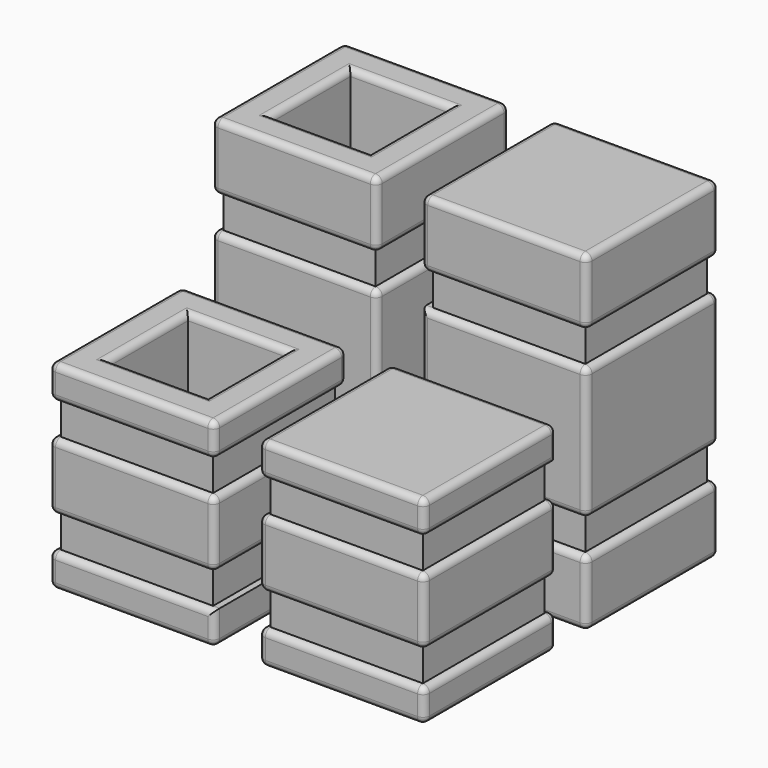
from build123d import *

# Parameters (mm, degrees)
F0_W     = 25
F0_H     = 25
F0_W_2   = 23
F0_H_2   = 23
F0_W_3   = 15
F0_H_3   = 15
F1_DEPTH = 50
F2_DEPTH = 30
F3_START = 20
F3_DEPTH = 5
F4_START = 5
F4_DEPTH = 5
F5_START = 35
F5_DEPTH = 5
F6_START = 10
F6_DEPTH = 5
F7_R     = 0.99999
F7_2_R   = 0.99999
F8_R     = 0.99999
F8_2_R   = 0.99999


# Not quite as in the source:
# - a fillet or chamfer is up to 0.001 mm smaller than in the source, because OpenCascade refuses the exact size


with BuildPart() as f1:
    # F0 (on Top) → F1 (new body)
    with BuildSketch(Plane.XY):
        with Locations((15.8383478876, 15.3343726881)):
            Rectangle(F0_W, F0_H)
        with Locations((15.8383478876, 15.3343726881)):
            Rectangle(F0_W_2, F0_H_2, mode=Mode.SUBTRACT)
        with Locations((15.8383478876, 15.3343726881)):
            Rectangle(F0_W_2, F0_H_2)
        with Locations((15.8383478876, 15.3343726881)):
            Rectangle(F0_W_3, F0_H_3, mode=Mode.SUBTRACT)
        with Locations((15.8383478876, 15.3343726881)):
            Rectangle(F0_W_3, F0_H_3)
    extrude(amount=F1_DEPTH)


with BuildPart() as f1b:
    # F0 (on Top) → F1, piece 2 (new body)
    with BuildSketch(Plane.XY):
        with Locations((-15.8383478876, 15.3343726881)):
            Rectangle(F0_W, F0_H)
        with Locations((-15.8383478876, 15.3343726881)):
            Rectangle(F0_W_2, F0_H_2, mode=Mode.SUBTRACT)
        with Locations((-15.8383478876, 15.3343726881)):
            Rectangle(F0_W_2, F0_H_2)
        with Locations((-15.8383478876, 15.3343726881)):
            Rectangle(F0_W_3, F0_H_3, mode=Mode.SUBTRACT)
    extrude(amount=F1_DEPTH)


with BuildPart() as f2:
    # F0 (on Top) → F2 (new body)
    with BuildSketch(Plane.XY):
        with Locations((-15.8383478876, -15.3343726881)):
            Rectangle(F0_W, F0_H)
        with Locations((-15.8383478876, -15.3343726881)):
            Rectangle(F0_W_2, F0_H_2, mode=Mode.SUBTRACT)
        with Locations((-15.8383478876, -15.3343726881)):
            Rectangle(F0_W_2, F0_H_2)
        with Locations((-15.8383478876, -15.3343726881)):
            Rectangle(F0_W_3, F0_H_3, mode=Mode.SUBTRACT)
    extrude(amount=F2_DEPTH)


with BuildPart() as f2b:
    # F0 (on Top) → F2, piece 2 (new body)
    with BuildSketch(Plane.XY):
        with Locations((15.8383478876, -15.3343726881)):
            Rectangle(F0_W, F0_H)
        with Locations((15.8383478876, -15.3343726881)):
            Rectangle(F0_W_2, F0_H_2, mode=Mode.SUBTRACT)
        with Locations((15.8383478876, -15.3343726881)):
            Rectangle(F0_W_2, F0_H_2)
        with Locations((15.8383478876, -15.3343726881)):
            Rectangle(F0_W_3, F0_H_3, mode=Mode.SUBTRACT)
        with Locations((15.8383478876, -15.3343726881)):
            Rectangle(F0_W_3, F0_H_3)
    extrude(amount=F2_DEPTH)


with BuildPart() as f3_tool:
    # F0 (on Top) → F3 (new body)
    with BuildSketch(Plane.XY.offset(F3_START)):
        with Locations((-15.8383478876, -15.3343726881)):
            Rectangle(F0_W, F0_H)
        with Locations((-15.8383478876, -15.3343726881)):
            Rectangle(F0_W_2, F0_H_2, mode=Mode.SUBTRACT)
        with Locations((15.8383478876, -15.3343726881)):
            Rectangle(F0_W, F0_H)
        with Locations((15.8383478876, -15.3343726881)):
            Rectangle(F0_W_2, F0_H_2, mode=Mode.SUBTRACT)
    extrude(amount=F3_DEPTH)


with BuildPart() as f2_1:
    add(f2.part)

    # F3: cut by f3_tool
    add(f3_tool.part, mode=Mode.SUBTRACT)


with BuildPart() as f2b_1:
    add(f2b.part)

    # F3: cut by f3_tool
    add(f3_tool.part, mode=Mode.SUBTRACT)


with BuildPart() as f4_tool:
    # F0 (on Top) → F4 (new body)
    with BuildSketch(Plane.XY.offset(F4_START)):
        with Locations((-15.8383478876, -15.3343726881)):
            Rectangle(F0_W, F0_H)
        with Locations((-15.8383478876, -15.3343726881)):
            Rectangle(F0_W_2, F0_H_2, mode=Mode.SUBTRACT)
        with Locations((15.8383478876, -15.3343726881)):
            Rectangle(F0_W, F0_H)
        with Locations((15.8383478876, -15.3343726881)):
            Rectangle(F0_W_2, F0_H_2, mode=Mode.SUBTRACT)
    extrude(amount=F4_DEPTH)


with BuildPart() as f2_2:
    add(f2_1.part)

    # F4: cut by f4_tool
    add(f4_tool.part, mode=Mode.SUBTRACT)

    # F8 (radius 1 in the source; OpenCascade refuses exactly that, so slightly less here)
    f8_edges = [f2_2.edges().sort_by_distance(p)[0] for p in [
        (-15.838348, -2.834373, 10),
        (-28.338348, -2.834373, 15),
        (-15.838348, -2.834373, 20),
        (-3.338348, -2.834373, 15),
        (-3.338348, -15.334373, 10),
        (-3.338348, -15.334373, 20),
        (-3.338348, -27.834373, 15),
        (-15.838348, -2.834373, 25),
        (-28.338348, -2.834373, 27.5),
        (-15.838348, -2.834373, 30),
        (-3.338348, -2.834373, 27.5),
        (-3.338348, -15.334373, 25),
        (-3.338348, -15.334373, 30),
        (-3.338348, -27.834373, 27.5),
        (-28.338348, -15.334373, 30),
        (-15.838348, -27.834373, 30),
        (-15.838348, -22.834373, 30),
        (-23.338348, -15.334373, 30),
        (-15.838348, -7.834373, 30),
        (-8.338348, -15.334373, 30),
        (-15.838348, -2.834373, 0),
        (-28.338348, -2.834373, 2.5),
        (-15.838348, -2.834373, 5),
        (-3.338348, -2.834373, 2.5),
        (-28.338348, -15.334373, 0),
        (-28.338348, -27.834373, 2.5),
        (-28.338348, -15.334373, 5),
        (-28.338348, -15.334373, 10),
        (-28.338348, -27.834373, 15),
        (-28.338348, -15.334373, 20),
        (-15.838348, -27.834373, 10),
        (-15.838348, -27.834373, 20),
        (-15.838348, -27.834373, 0),
        (-3.338348, -27.834373, 2.5),
        (-15.838348, -27.834373, 5),
        (-3.338348, -15.334373, 0),
        (-15.838348, -22.834373, 0),
        (-23.338348, -15.334373, 0),
        (-15.838348, -7.834373, 0),
        (-8.338348, -15.334373, 0),
        (-28.338348, -15.334373, 25),
        (-28.338348, -27.834373, 27.5),
        (-15.838348, -27.834373, 25),
    ]]
    fillet(f8_edges, radius=F8_R)


with BuildPart() as f2b_2:
    add(f2b_1.part)

    # F4: cut by f4_tool
    add(f4_tool.part, mode=Mode.SUBTRACT)

    # F8#2 (radius 1 in the source; OpenCascade refuses exactly that, so slightly less here)
    f8_2_edges = [f2b_2.edges().sort_by_distance(p)[0] for p in [
        (15.838348, -27.834373, 0),
        (28.338348, -15.334373, 0),
        (15.838348, -2.834373, 0),
        (3.338348, -15.334373, 0),
        (28.338348, -2.834373, 2.5),
        (28.338348, -15.334373, 5),
        (28.338348, -27.834373, 2.5),
        (15.838348, -27.834373, 5),
        (3.338348, -27.834373, 2.5),
        (28.338348, -15.334373, 10),
        (28.338348, -2.834373, 15),
        (28.338348, -15.334373, 20),
        (28.338348, -27.834373, 15),
        (15.838348, -27.834373, 10),
        (15.838348, -27.834373, 20),
        (3.338348, -27.834373, 15),
        (28.338348, -15.334373, 25),
        (28.338348, -2.834373, 27.5),
        (28.338348, -15.334373, 30),
        (28.338348, -27.834373, 27.5),
        (15.838348, -27.834373, 25),
        (15.838348, -27.834373, 30),
        (3.338348, -27.834373, 27.5),
        (15.838348, -2.834373, 30),
        (3.338348, -15.334373, 30),
        (3.338348, -15.334373, 5),
        (3.338348, -2.834373, 2.5),
        (15.838348, -2.834373, 5),
        (15.838348, -2.834373, 10),
        (3.338348, -2.834373, 15),
        (15.838348, -2.834373, 20),
        (3.338348, -15.334373, 10),
        (3.338348, -15.334373, 20),
        (3.338348, -15.334373, 25),
        (3.338348, -2.834373, 27.5),
    ]]
    fillet(f8_2_edges, radius=F8_2_R)


with BuildPart() as f5_tool:
    # F0 (on Top) → F5 (new body)
    with BuildSketch(Plane.XY.offset(F5_START)):
        with Locations((15.8383478876, 15.3343726881)):
            Rectangle(F0_W, F0_H)
        with Locations((15.8383478876, 15.3343726881)):
            Rectangle(F0_W_2, F0_H_2, mode=Mode.SUBTRACT)
        with Locations((-15.8383478876, 15.3343726881)):
            Rectangle(F0_W, F0_H)
        with Locations((-15.8383478876, 15.3343726881)):
            Rectangle(F0_W_2, F0_H_2, mode=Mode.SUBTRACT)
    extrude(amount=F5_DEPTH)


with BuildPart() as f1_1:
    add(f1.part)

    # F5: cut by f5_tool
    add(f5_tool.part, mode=Mode.SUBTRACT)


with BuildPart() as f1b_1:
    add(f1b.part)

    # F5: cut by f5_tool
    add(f5_tool.part, mode=Mode.SUBTRACT)


with BuildPart() as f6_tool:
    # F0 (on Top) → F6 (new body)
    with BuildSketch(Plane.XY.offset(F6_START)):
        with Locations((15.8383478876, 15.3343726881)):
            Rectangle(F0_W, F0_H)
        with Locations((15.8383478876, 15.3343726881)):
            Rectangle(F0_W_2, F0_H_2, mode=Mode.SUBTRACT)
        with Locations((-15.8383478876, 15.3343726881)):
            Rectangle(F0_W, F0_H)
        with Locations((-15.8383478876, 15.3343726881)):
            Rectangle(F0_W_2, F0_H_2, mode=Mode.SUBTRACT)
    extrude(amount=F6_DEPTH)


with BuildPart() as f1_2:
    add(f1_1.part)

    # F6: cut by f6_tool
    add(f6_tool.part, mode=Mode.SUBTRACT)

    # F7 (radius 1 in the source; OpenCascade refuses exactly that, so slightly less here)
    f7_edges = [f1_2.edges().sort_by_distance(p)[0] for p in [
        (15.838348, 27.834373, 40),
        (3.338348, 27.834373, 45),
        (15.838348, 27.834373, 50),
        (28.338348, 27.834373, 45),
        (28.338348, 15.334373, 40),
        (28.338348, 15.334373, 50),
        (28.338348, 2.834373, 45),
        (15.838348, 2.834373, 40),
        (15.838348, 2.834373, 50),
        (3.338348, 2.834373, 45),
        (3.338348, 15.334373, 40),
        (3.338348, 15.334373, 50),
        (3.338348, 2.834373, 25),
        (15.838348, 2.834373, 15),
        (28.338348, 2.834373, 25),
        (15.838348, 2.834373, 35),
        (28.338348, 15.334373, 15),
        (28.338348, 27.834373, 25),
        (28.338348, 15.334373, 35),
        (15.838348, 27.834373, 15),
        (3.338348, 27.834373, 25),
        (15.838348, 27.834373, 35),
        (28.338348, 15.334373, 0),
        (28.338348, 27.834373, 5),
        (28.338348, 15.334373, 10),
        (28.338348, 2.834373, 5),
        (15.838348, 27.834373, 0),
        (3.338348, 27.834373, 5),
        (15.838348, 27.834373, 10),
        (15.838348, 2.834373, 0),
        (15.838348, 2.834373, 10),
        (3.338348, 2.834373, 5),
        (3.338348, 15.334373, 0),
        (3.338348, 15.334373, 10),
    ]]
    fillet(f7_edges, radius=F7_R)


with BuildPart() as f1b_2:
    add(f1b_1.part)

    # F6: cut by f6_tool
    add(f6_tool.part, mode=Mode.SUBTRACT)

    # F7#2 (radius 1 in the source; OpenCascade refuses exactly that, so slightly less here)
    f7_2_edges = [f1b_2.edges().sort_by_distance(p)[0] for p in [
        (-3.338348, 15.334373, 0),
        (-15.838348, 27.834373, 0),
        (-28.338348, 15.334373, 0),
        (-15.838348, 2.834373, 0),
        (-15.838348, 7.834373, 0),
        (-23.338348, 15.334373, 0),
        (-15.838348, 22.834373, 0),
        (-8.338348, 15.334373, 0),
        (-28.338348, 2.834373, 5),
        (-28.338348, 15.334373, 10),
        (-28.338348, 27.834373, 5),
        (-3.338348, 27.834373, 5),
        (-3.338348, 15.334373, 10),
        (-3.338348, 2.834373, 5),
        (-15.838348, 27.834373, 10),
        (-15.838348, 2.834373, 10),
        (-15.838348, 2.834373, 15),
        (-3.338348, 2.834373, 25),
        (-15.838348, 2.834373, 35),
        (-28.338348, 2.834373, 25),
        (-28.338348, 15.334373, 15),
        (-28.338348, 15.334373, 35),
        (-28.338348, 27.834373, 25),
        (-15.838348, 2.834373, 40),
        (-3.338348, 2.834373, 45),
        (-15.838348, 2.834373, 50),
        (-28.338348, 2.834373, 45),
        (-28.338348, 15.334373, 40),
        (-28.338348, 15.334373, 50),
        (-28.338348, 27.834373, 45),
        (-3.338348, 15.334373, 50),
        (-15.838348, 27.834373, 50),
        (-15.838348, 7.834373, 50),
        (-23.338348, 15.334373, 50),
        (-15.838348, 22.834373, 50),
        (-8.338348, 15.334373, 50),
        (-15.838348, 27.834373, 15),
        (-15.838348, 27.834373, 35),
        (-3.338348, 27.834373, 25),
        (-3.338348, 15.334373, 15),
        (-3.338348, 15.334373, 35),
        (-15.838348, 27.834373, 40),
        (-3.338348, 27.834373, 45),
        (-3.338348, 15.334373, 40),
    ]]
    fillet(f7_2_edges, radius=F7_2_R)


solid = Compound([f2_2.part, f2b_2.part, f1_2.part, f1b_2.part])
